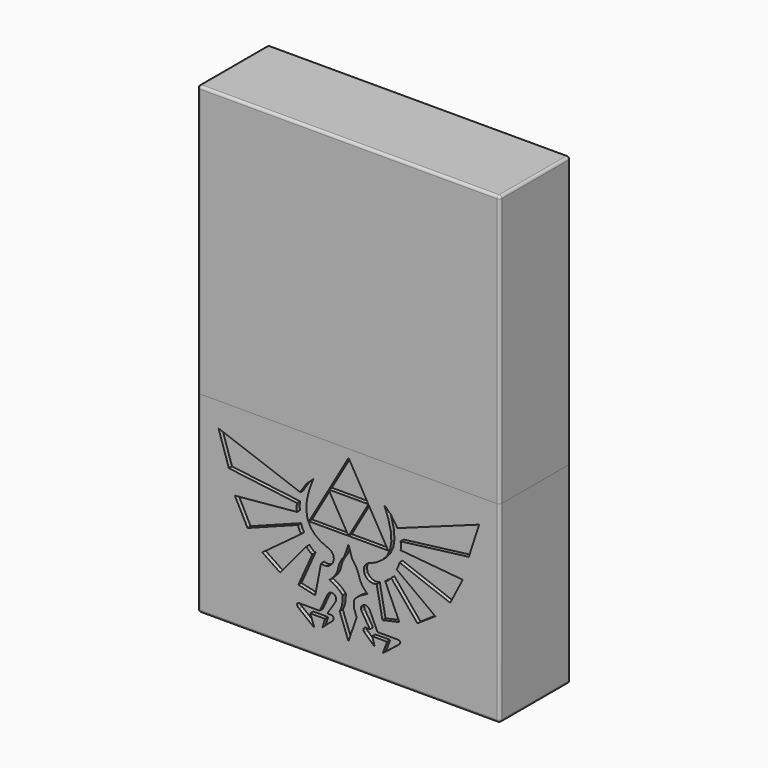
from build123d import *

# Parameters (mm, degrees)
F3_DEPTH  = 1.5
F4_W      = 58
F4_H      = 17
F6_DEPTH  = 35.5
F7_W      = 55
F7_H      = 14
F9_DEPTH  = 15
F8_W      = 58
F8_H      = 17
F10_DEPTH = 15
F11_W     = 58
F11_H     = 17
F11_W_2   = 55
F11_H_2   = 14
F12_DEPTH = 35.5
F13_W     = 58
F13_H     = 17
F14_DEPTH = 1.5
F15_R     = 0.5
F15_2_R   = 0.5
F17_DEPTH = 0.75


# Not quite as in the source:
# - a pattern or mirror of a feature is missing from the dataset's text; its kind, count and spacing are read off the source's solid


with BuildPart() as f3:
    # F1 (on Top) → F3 (new body)
    with BuildSketch(Plane.XY):
        Polygon((-29, 8.5), (-29, 0), (-29, -8.5), (0, -8.5), (29, -8.5), (29, 0), (29, 8.5), (0, 8.5), align=None)
    extrude(amount=F3_DEPTH)

    # F4 (on face) → F6 (join)
    with BuildSketch(Plane.XY.offset(1.5)):
        Rectangle(F4_W, F4_H)
        Polygon((-27.5, -7), (-27.5, 0), (-27.5, 7), (0, 7), (27.5, 7), (27.5, 0), (27.5, -7), (0, -7), align=None, mode=Mode.SUBTRACT)
    extrude(amount=F6_DEPTH)

    # F7 (on face) → F9 (join)
    with BuildSketch(Plane.XY.offset(37)):
        Polygon((-28.15, 7.65), (-28.15, 0), (-28.15, -7.65), (0, -7.65), (28.15, -7.65), (28.15, 0), (28.15, 7.65), (0, 7.65), align=None)
        Rectangle(F7_W, F7_H, mode=Mode.SUBTRACT)
    extrude(amount=F9_DEPTH)

    # F15
    f15_edges = [f3.edges().sort_by_distance(p)[0] for p in [
        (-29, -8.5, 18.5),
        (-29, 8.5, 18.5),
        (29, 8.5, 18.5),
        (29, -8.5, 18.5),
        (28.15, -7.65, 44.5),
        (28.15, 7.65, 44.5),
        (-28.15, 7.65, 44.5),
        (-28.15, -7.65, 44.5),
        (27.5, 7, 26.75),
        (-27.5, 7, 26.75),
        (-27.5, -7, 26.75),
        (27.5, -7, 26.75),
        (-29, 0, 0),
        (0, -8.5, 0),
        (29, 0, 0),
        (0, 8.5, 0),
    ]]
    fillet(f15_edges, radius=F15_R)

    # F16 (on face) → F17 (cut)
    with BuildSketch(Plane.XZ.offset(8.5)):
        Polygon((-24.9505469647, 32.3474604987), (-22.9699474098, 26.261089324), (-9.8792146069, 24.6190482749), (-9.8929405752, 24.5376152192), (-9.9373481197, 24.2929700193), (-9.9780646476, 23.9518970085), (-9.9692984829, 23.5707995354), (-9.9110496258, 23.2316873772), (-9.8792146069, 23.1214182536), (-21.8103683795, 22.0101915419), (-19.3954745735, 17.3249072333), (-9.6857822636, 20.995738674), (-9.6570615399, 20.8687446311), (-9.4643212623, 20.269300452), (-9.1808050429, 19.7366406062), (-9.1062926435, 19.6434424348), (-16.5456521229, 14.136526277), (-13.1157748654, 11.8180141443), (-8.0919551199, 17.8561829478), (-8.0343983284, 17.7935510084), (-7.8661110363, 17.599657288), (-7.6257335744, 17.3486681532), (-7.3290681081, 17.122132004), (-7.0362090028, 16.9732225494), (-6.933091224, 16.9381578909), (-9.6376837023, 10.8999890873), (-6.4010080996, 10.1753156327), (-5.2903581092, 15.9238203673), (-5.1112284556, 15.8568053455), (-4.5225112938, 15.7897903238), (-3.8610118967, 15.9475812872), (-3.3372335598, 16.3242956779), (-2.9812811379, 16.8480740149), (-2.8234901745, 17.4462494069), (-2.8936194916, 18.0470777172), (-3.2226966982, 18.5783534317), (-3.6739234883, 18.9037396217), (-3.8410573377, 18.9669482824), (-4.2170796628, 19.0939423254), (-5.3015465036, 19.5996116117), (-6.4699839739, 20.4206321363), (-7.3340279118, 21.4376225781), (-7.8854888739, 22.6565808394), (-8.1120250231, 24.0845429207), (-8.0037167522, 25.7285448225), (-7.5499523881, 27.5952765126), (-6.9693093253, 29.1790687046), (-6.7396588807, 29.6909665816), (-6.9673484727, 29.5225639452), (-8.063119052, 28.4906940923), (-9.0694978209, 27.0307816478), (-9.2515110813, 26.6478386664), align=None)
        Polygon((-3.810045387, 28.8679168418), (-7.6046381146, 22.2954894436), (-0.0154526594, 22.2954894436), align=None)
        Polygon((3.810045387, 28.8679168418), (0.0154526594, 22.2954894436), (7.6046381146, 22.2954894436), align=None)
        Polygon((0, 35.4671090312), (-3.7945927276, 28.894681633), (3.7945927276, 28.894681633), align=None)
        Polygon((-4.5174361458, 6.8186243155), (-5.0006132992, 5.2003557206), (-3.0682507186, 6.9394013021), (-3.0061955006, 6.9994725988), (-2.87170408, 7.2353977717), (-2.8434447335, 7.5389031533), (-2.9999669099, 7.7723138211), (-3.2696418167, 7.8599293298), (-3.3578801844, 7.8568035), (-4.0825882423, 7.8568035), (-2.4886457543, 10.3687018383), (-2.4405471931, 10.4631803311), (-2.3622284327, 10.7810806778), (-2.4079047642, 11.1246335905), (-2.5857656309, 11.3887258346), (-2.8553251934, 11.5626880648), (-3.1757515797, 11.635897074), (-3.5062129175, 11.597095261), (-3.8059926792, 11.4362707433), (-3.9943498746, 11.2235067001), (-4.0343743368, 11.1415315263), (-5.5317736695, 7.8568035), (-9.3479388923, 7.8568035), (-9.4517487367, 7.8605521888), (-9.7652544666, 7.7879660388), (-9.9154327081, 7.5777049662), (-9.8185435201, 7.2779482735), (-9.5843946489, 7.0113645931), (-9.4930419859, 6.9394013021), (-6.5463418817, 4.6202547759), (-7.3673624063, 6.8186243155), align=None)
        Polygon((-1.7158391352, 9.0507897265), (-0.0248921149, 4.4756938005), (1.5575159459, 9.0507897265), (1.450476462, 9.255433533), (1.0864499411, 10.3549181979), (1.0431958393, 11.598364048), (1.0964848927, 11.8749480767), (1.2102143444, 12.0439159), (1.6407945099, 12.4907250045), (2.2710356095, 12.9469115984), (2.9455689092, 13.3186200477), (3.4574667862, 13.5864609806), (3.6246006356, 13.6822197948), (3.4806509848, 13.8054882177), (3.0770613787, 14.2072438498), (2.6164917026, 14.7835961057), (2.2584630839, 15.4200081237), (2.0613397239, 15.9450437132), (2.0187776877, 16.1253268096), (1.9556843712, 16.3637434188), (1.5037655154, 17.4619362278), (0.8586450048, 18.4312894856), (0.6997005987, 18.6046519256), (-0.0248921149, 20.8510969575), (-0.7979294225, 18.6046519256), (-0.9079678576, 18.4744282431), (-1.2108619145, 18.0620724725), (-1.5588555817, 17.4738166878), (-1.8278384228, 16.8311184069), (-1.974902369, 16.3042257747), (-2.0055839452, 16.1253268096), (-2.0418020465, 15.9324711876), (-2.2521899977, 15.372463215), (-2.6444758651, 14.73478241), (-3.1283450841, 14.1822141429), (-3.5161325249, 13.8048653587), (-3.64831706, 13.6822197948), (-3.4825673419, 13.598352975), (-2.9849721546, 13.3436612891), (-2.3341997748, 12.9656896458), (-1.7121481185, 12.4944736934), (-1.2647276893, 12.0420357884), (-1.1363495151, 11.8749480767), (-1.1288521375, 11.6340284968), (-1.1557273528, 10.9081208585), (-1.2702642144, 10.1384054658), (-1.4624277707, 9.5313947026), (-1.6425955228, 9.1640578011), align=None)
        Polygon((9.978109143, 24.6190482749), (23.0688765492, 26.261089324), (25.0494530353, 32.3474604987), (9.3505209618, 26.6478386664), (9.1683923571, 27.0307816478), (8.1621289324, 28.4906940923), (7.0656662875, 29.5225639452), (6.8385534169, 29.6909665816), (7.0676271401, 29.1797607703), (7.6483855471, 27.5952765126), (8.1027266326, 25.7285448225), (8.2110349035, 24.0845429207), (7.9844987543, 22.6565808394), (7.4330377922, 21.4376225781), (6.5689938544, 20.4206321363), (5.400556384, 19.5996116117), (4.3160895433, 19.0939423254), (3.9405285953, 18.9669482824), (3.7729333688, 18.9037396217), (3.3217065786, 18.5783534317), (2.9925140277, 18.0470777172), (2.9218079893, 17.4462494069), (3.0800603298, 16.8480740149), (3.4362434402, 16.3242956779), (3.9600217771, 15.9475812872), (4.6209444529, 15.7897903238), (5.2096616147, 15.8568053455), (5.3892526454, 15.9238203673), (6.5007100456, 10.1753156327), (9.7372703041, 10.8999890873), (7.0318704159, 16.9381578909), (7.1346421618, 16.9732225494), (7.4275012672, 17.122132004), (7.7241667335, 17.3486681532), (7.9644288511, 17.599657288), (8.1326007989, 17.7935510084), (8.1909650003, 17.8561829478), (13.2146694015, 11.8180141443), (16.6445466591, 14.136526277), (9.2053025239, 19.6434424348), (9.279238202, 19.7366406062), (9.5632157984, 20.269300452), (9.7559560761, 20.8687446311), (9.7854842096, 20.995738674), (19.4943575752, 17.3249072333), (21.9098973091, 22.0101915419), (9.978109143, 23.1214182536), (10.0093674406, 23.2316873772), (10.067731642, 23.5707995354), (10.0763824624, 23.9518970085), (10.0356659345, 24.2929700193), (9.9919504556, 24.5376152192), align=None)
        Polygon((3.0889418387, 6.9394013021), (5.0207276979, 5.2003557206), (4.5375505446, 6.8186243155), (7.3880535263, 6.8186243155), (6.5670330018, 4.6202547759), (9.5132717289, 6.9394013021), (9.6039323263, 7.0113645931), (9.8379658532, 7.2779482735), (9.9355471069, 7.5777049662), (9.7854842096, 7.7879660388), (9.4719784797, 7.8605521888), (9.3686300124, 7.8568035), (5.5520034125, 7.8568035), (4.0550654569, 11.1415315263), (4.014348929, 11.2235067001), (3.8261070779, 11.4362707433), (3.5257505949, 11.597095261), (3.195289257, 11.635897074), (2.8755549364, 11.5626880648), (2.6057646854, 11.3887258346), (2.4274424416, 11.1246335905), (2.3817661101, 10.7810806778), (2.4599695262, 10.4631803311), (2.508760153, 10.3687018383), (4.1032793624, 7.8568035), (3.3786866487, 7.8568035), (3.2897562154, 7.8599293298), (3.0199659644, 7.7723138211), (2.8629824108, 7.5389031533), (2.8918184787, 7.2353977717), (3.0263098993, 6.9994725988), align=None)
    f17 = extrude(amount=-F17_DEPTH, mode=Mode.SUBTRACT)

    # F17_copies: F17 across plane
    add(f17.mirror(Plane.ZX), mode=Mode.SUBTRACT)


with BuildPart() as f10:
    # F8 (on face) → F10 (new body, through all)
    with BuildSketch(Plane.XY.offset(37)):
        Rectangle(F8_W, F8_H)
        Polygon((-28.35, -7.85), (-28.35, 0), (-28.35, 7.85), (0, 7.85), (28.35, 7.85), (28.35, 0), (28.35, -7.85), (0, -7.85), align=None, mode=Mode.SUBTRACT)
    extrude(amount=F10_DEPTH)

    # F11 (on face) → F12 (join)
    with BuildSketch(Plane.XY.offset(52)):
        Rectangle(F11_W, F11_H)
        Rectangle(F11_W_2, F11_H_2, mode=Mode.SUBTRACT)
    extrude(amount=F12_DEPTH)

    # F13 (on face) → F14 (join)
    with BuildSketch(Plane.XY.offset(87.5)):
        Rectangle(F13_W, F13_H)
    extrude(amount=F14_DEPTH)

    # F15#2
    f15_2_edges = [f10.edges().sort_by_distance(p)[0] for p in [
        (-29, -8.5, 63),
        (-29, 8.5, 63),
        (29, -8.5, 63),
        (29, 8.5, 63),
        (-28.35, -7.85, 44.5),
        (-28.35, 7.85, 44.5),
        (28.35, 7.85, 44.5),
        (28.35, -7.85, 44.5),
        (27.5, -7, 69.75),
        (27.5, 7, 69.75),
        (-27.5, -7, 69.75),
        (-27.5, 7, 69.75),
        (0, 8.5, 89),
        (-29, 0, 89),
        (0, -8.5, 89),
        (29, 0, 89),
    ]]
    fillet(f15_2_edges, radius=F15_2_R)


solid = Compound([f3.part, f10.part])
